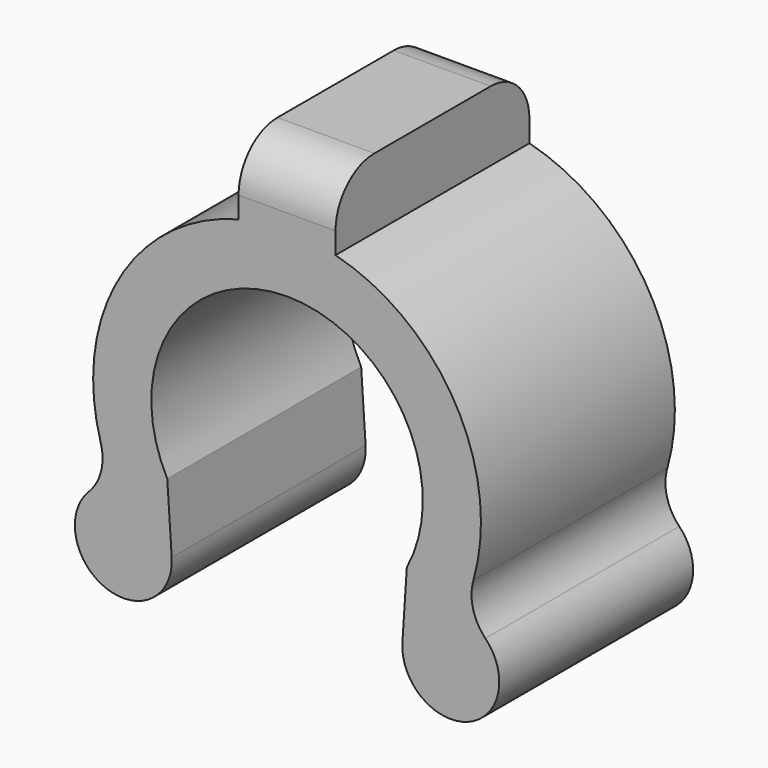
from build123d import *

# Parameters (mm, degrees)
F1_DEPTH = 25
F3_R     = 5


# Not quite as in the source:
# - a feature names something its author has since deleted; it is built from what else it names


with BuildPart() as f1:
    # F0 (on Front) → F1 (new body)
    with BuildSketch(Plane.XZ):
        with BuildLine():
            ThreePointArc((11.897, -13.5710131507), (19.9295853554, -17.8647399206), (17.8635986234, -8.9939893385))
            ThreePointArc((17.8635986234, -8.9939893385), (18.2138113493, 8.2617840768), (5, 19.364916731))
            Line((5, 19.364916731), (5, 26.5722312033))
            Line((5, 26.5722312033), (0, 26.5722312033))
            Line((0, 26.5722312033), (0, 20))
            Line((0, 20), (0, 14))
            ThreePointArc((0, 14), (12.0042367313, 7.2040475081), (12.3541559587, -6.5859570715))
            Line((12.3541559587, -6.5859570715), (11.897, -13.5710131507))
        make_face()
    extrude(amount=F1_DEPTH)

    # F2: F1 across plane


with BuildPart() as f1_1:
    add(f1.part)
    add(f1.part.mirror(Plane.YZ))

    # F3
    f3_edges = [f1_1.edges().sort_by_distance(p)[0] for p in [
        (-17.863599, -12.5, -8.993989),
        (17.863599, -12.5, -8.993989),
        (0, -25, 26.572231),
        (0, 0, 26.572231),
    ]]
    fillet(f3_edges, radius=F3_R)


solid = f1_1.part
